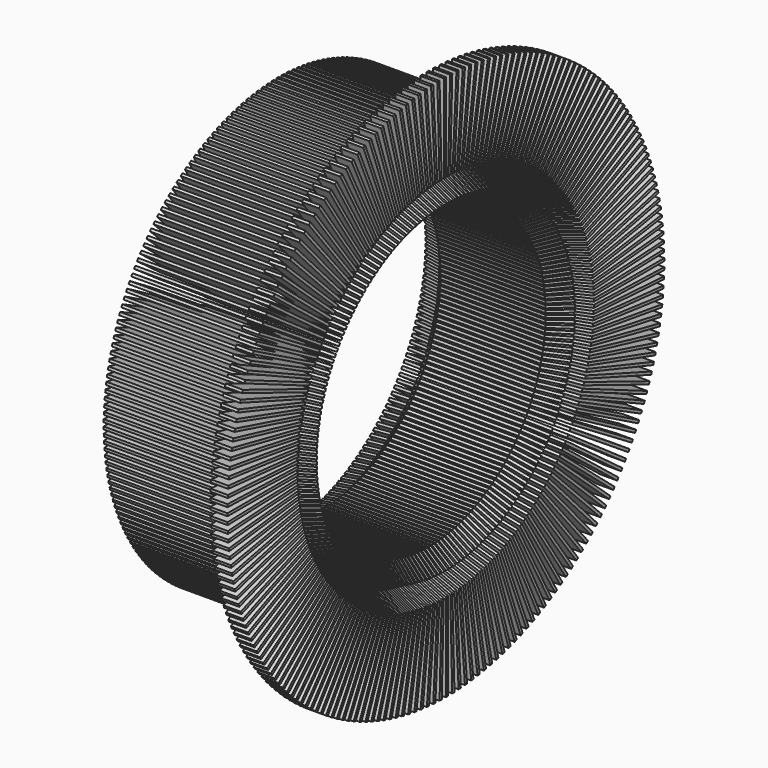
from build123d import *

# Parameters (mm, degrees)
F0_R     = 13
F1_DEPTH = 3
F2_COUNT = 216
F2_ANGLE = 358.333319


with BuildPart() as f1:
    # F0 (on Front) → F1 (new body)
    with BuildSketch(Plane.XZ):
        with BuildLine():
            Line((79.4218590744, 204.5887249741), (79.4218590744, 302.0993764614))
            Line((79.4218590744, 302.0993764614), (60.4218590744, 302.0993764614))
            Line((60.4218590744, 302.0993764614), (60.4218590744, 242.0993764614))
            ThreePointArc((60.4218590744, 242.0993764614), (55.8752099476, 238.8486342481), (51.3285608207, 242.0993764614))
            Line((51.3285608207, 242.0993764614), (-105.6314391793, 242.0993764614))
            Line((-105.6314391793, 242.0993764614), (-105.6314391793, 202.8593764614))
            Line((-105.6314391793, 202.8593764614), (-56.7432582628, 192.3738737706))
            Line((-56.7432582628, 192.3738737706), (-70.0419396162, 177.6219755411))
            Line((-70.0419396162, 177.6219755411), (-56.2349801763, 162))
            Line((-56.2349801763, 162), (60.158367424, 162))
            Line((60.158367424, 162), (79.4218590744, 178.5993582789))
            Line((79.4218590744, 178.5993582789), (52.476448941, 192.3738737706))
            Line((52.476448941, 192.3738737706), (79.4218590744, 204.5887249741))
        make_face()
        with Locations((5.6830663262, 192.3738737706)):
            Circle(F0_R, mode=Mode.SUBTRACT)
    extrude(amount=F1_DEPTH)


with BuildPart() as f2_1:
    # F2: instance of F1
    add(f1.part.rotate(Axis((24.8979143798, 0, 0), (1, 0, 0)), 1 * F2_ANGLE / (F2_COUNT - 1)))


with BuildPart() as f2_2:
    # F2: instance of F1
    add(f1.part.rotate(Axis((24.8979143798, 0, 0), (1, 0, 0)), 2 * F2_ANGLE / (F2_COUNT - 1)))


with BuildPart() as f2_3:
    # F2: instance of F1
    add(f1.part.rotate(Axis((24.8979143798, 0, 0), (1, 0, 0)), 3 * F2_ANGLE / (F2_COUNT - 1)))


with BuildPart() as f2_4:
    # F2: instance of F1
    add(f1.part.rotate(Axis((24.8979143798, 0, 0), (1, 0, 0)), 4 * F2_ANGLE / (F2_COUNT - 1)))


with BuildPart() as f2_5:
    # F2: instance of F1
    add(f1.part.rotate(Axis((24.8979143798, 0, 0), (1, 0, 0)), 5 * F2_ANGLE / (F2_COUNT - 1)))


with BuildPart() as f2_6:
    # F2: instance of F1
    add(f1.part.rotate(Axis((24.8979143798, 0, 0), (1, 0, 0)), 6 * F2_ANGLE / (F2_COUNT - 1)))


with BuildPart() as f2_7:
    # F2: instance of F1
    add(f1.part.rotate(Axis((24.8979143798, 0, 0), (1, 0, 0)), 7 * F2_ANGLE / (F2_COUNT - 1)))


with BuildPart() as f2_8:
    # F2: instance of F1
    add(f1.part.rotate(Axis((24.8979143798, 0, 0), (1, 0, 0)), 8 * F2_ANGLE / (F2_COUNT - 1)))


with BuildPart() as f2_9:
    # F2: instance of F1
    add(f1.part.rotate(Axis((24.8979143798, 0, 0), (1, 0, 0)), 9 * F2_ANGLE / (F2_COUNT - 1)))


with BuildPart() as f2_10:
    # F2: instance of F1
    add(f1.part.rotate(Axis((24.8979143798, 0, 0), (1, 0, 0)), 10 * F2_ANGLE / (F2_COUNT - 1)))


with BuildPart() as f2_11:
    # F2: instance of F1
    add(f1.part.rotate(Axis((24.8979143798, 0, 0), (1, 0, 0)), 11 * F2_ANGLE / (F2_COUNT - 1)))


with BuildPart() as f2_12:
    # F2: instance of F1
    add(f1.part.rotate(Axis((24.8979143798, 0, 0), (1, 0, 0)), 12 * F2_ANGLE / (F2_COUNT - 1)))


with BuildPart() as f2_13:
    # F2: instance of F1
    add(f1.part.rotate(Axis((24.8979143798, 0, 0), (1, 0, 0)), 13 * F2_ANGLE / (F2_COUNT - 1)))


with BuildPart() as f2_14:
    # F2: instance of F1
    add(f1.part.rotate(Axis((24.8979143798, 0, 0), (1, 0, 0)), 14 * F2_ANGLE / (F2_COUNT - 1)))


with BuildPart() as f2_15:
    # F2: instance of F1
    add(f1.part.rotate(Axis((24.8979143798, 0, 0), (1, 0, 0)), 15 * F2_ANGLE / (F2_COUNT - 1)))


with BuildPart() as f2_16:
    # F2: instance of F1
    add(f1.part.rotate(Axis((24.8979143798, 0, 0), (1, 0, 0)), 16 * F2_ANGLE / (F2_COUNT - 1)))


with BuildPart() as f2_17:
    # F2: instance of F1
    add(f1.part.rotate(Axis((24.8979143798, 0, 0), (1, 0, 0)), 17 * F2_ANGLE / (F2_COUNT - 1)))


with BuildPart() as f2_18:
    # F2: instance of F1
    add(f1.part.rotate(Axis((24.8979143798, 0, 0), (1, 0, 0)), 18 * F2_ANGLE / (F2_COUNT - 1)))


with BuildPart() as f2_19:
    # F2: instance of F1
    add(f1.part.rotate(Axis((24.8979143798, 0, 0), (1, 0, 0)), 19 * F2_ANGLE / (F2_COUNT - 1)))


with BuildPart() as f2_20:
    # F2: instance of F1
    add(f1.part.rotate(Axis((24.8979143798, 0, 0), (1, 0, 0)), 20 * F2_ANGLE / (F2_COUNT - 1)))


with BuildPart() as f2_21:
    # F2: instance of F1
    add(f1.part.rotate(Axis((24.8979143798, 0, 0), (1, 0, 0)), 21 * F2_ANGLE / (F2_COUNT - 1)))


with BuildPart() as f2_22:
    # F2: instance of F1
    add(f1.part.rotate(Axis((24.8979143798, 0, 0), (1, 0, 0)), 22 * F2_ANGLE / (F2_COUNT - 1)))


with BuildPart() as f2_23:
    # F2: instance of F1
    add(f1.part.rotate(Axis((24.8979143798, 0, 0), (1, 0, 0)), 23 * F2_ANGLE / (F2_COUNT - 1)))


with BuildPart() as f2_24:
    # F2: instance of F1
    add(f1.part.rotate(Axis((24.8979143798, 0, 0), (1, 0, 0)), 24 * F2_ANGLE / (F2_COUNT - 1)))


with BuildPart() as f2_25:
    # F2: instance of F1
    add(f1.part.rotate(Axis((24.8979143798, 0, 0), (1, 0, 0)), 25 * F2_ANGLE / (F2_COUNT - 1)))


with BuildPart() as f2_26:
    # F2: instance of F1
    add(f1.part.rotate(Axis((24.8979143798, 0, 0), (1, 0, 0)), 26 * F2_ANGLE / (F2_COUNT - 1)))


with BuildPart() as f2_27:
    # F2: instance of F1
    add(f1.part.rotate(Axis((24.8979143798, 0, 0), (1, 0, 0)), 27 * F2_ANGLE / (F2_COUNT - 1)))


with BuildPart() as f2_28:
    # F2: instance of F1
    add(f1.part.rotate(Axis((24.8979143798, 0, 0), (1, 0, 0)), 28 * F2_ANGLE / (F2_COUNT - 1)))


with BuildPart() as f2_29:
    # F2: instance of F1
    add(f1.part.rotate(Axis((24.8979143798, 0, 0), (1, 0, 0)), 29 * F2_ANGLE / (F2_COUNT - 1)))


with BuildPart() as f2_30:
    # F2: instance of F1
    add(f1.part.rotate(Axis((24.8979143798, 0, 0), (1, 0, 0)), 30 * F2_ANGLE / (F2_COUNT - 1)))


with BuildPart() as f2_31:
    # F2: instance of F1
    add(f1.part.rotate(Axis((24.8979143798, 0, 0), (1, 0, 0)), 31 * F2_ANGLE / (F2_COUNT - 1)))


with BuildPart() as f2_32:
    # F2: instance of F1
    add(f1.part.rotate(Axis((24.8979143798, 0, 0), (1, 0, 0)), 32 * F2_ANGLE / (F2_COUNT - 1)))


with BuildPart() as f2_33:
    # F2: instance of F1
    add(f1.part.rotate(Axis((24.8979143798, 0, 0), (1, 0, 0)), 33 * F2_ANGLE / (F2_COUNT - 1)))


with BuildPart() as f2_34:
    # F2: instance of F1
    add(f1.part.rotate(Axis((24.8979143798, 0, 0), (1, 0, 0)), 34 * F2_ANGLE / (F2_COUNT - 1)))


with BuildPart() as f2_35:
    # F2: instance of F1
    add(f1.part.rotate(Axis((24.8979143798, 0, 0), (1, 0, 0)), 35 * F2_ANGLE / (F2_COUNT - 1)))


with BuildPart() as f2_36:
    # F2: instance of F1
    add(f1.part.rotate(Axis((24.8979143798, 0, 0), (1, 0, 0)), 36 * F2_ANGLE / (F2_COUNT - 1)))


with BuildPart() as f2_37:
    # F2: instance of F1
    add(f1.part.rotate(Axis((24.8979143798, 0, 0), (1, 0, 0)), 37 * F2_ANGLE / (F2_COUNT - 1)))


with BuildPart() as f2_38:
    # F2: instance of F1
    add(f1.part.rotate(Axis((24.8979143798, 0, 0), (1, 0, 0)), 38 * F2_ANGLE / (F2_COUNT - 1)))


with BuildPart() as f2_39:
    # F2: instance of F1
    add(f1.part.rotate(Axis((24.8979143798, 0, 0), (1, 0, 0)), 39 * F2_ANGLE / (F2_COUNT - 1)))


with BuildPart() as f2_40:
    # F2: instance of F1
    add(f1.part.rotate(Axis((24.8979143798, 0, 0), (1, 0, 0)), 40 * F2_ANGLE / (F2_COUNT - 1)))


with BuildPart() as f2_41:
    # F2: instance of F1
    add(f1.part.rotate(Axis((24.8979143798, 0, 0), (1, 0, 0)), 41 * F2_ANGLE / (F2_COUNT - 1)))


with BuildPart() as f2_42:
    # F2: instance of F1
    add(f1.part.rotate(Axis((24.8979143798, 0, 0), (1, 0, 0)), 42 * F2_ANGLE / (F2_COUNT - 1)))


with BuildPart() as f2_43:
    # F2: instance of F1
    add(f1.part.rotate(Axis((24.8979143798, 0, 0), (1, 0, 0)), 43 * F2_ANGLE / (F2_COUNT - 1)))


with BuildPart() as f2_44:
    # F2: instance of F1
    add(f1.part.rotate(Axis((24.8979143798, 0, 0), (1, 0, 0)), 44 * F2_ANGLE / (F2_COUNT - 1)))


with BuildPart() as f2_45:
    # F2: instance of F1
    add(f1.part.rotate(Axis((24.8979143798, 0, 0), (1, 0, 0)), 45 * F2_ANGLE / (F2_COUNT - 1)))


with BuildPart() as f2_46:
    # F2: instance of F1
    add(f1.part.rotate(Axis((24.8979143798, 0, 0), (1, 0, 0)), 46 * F2_ANGLE / (F2_COUNT - 1)))


with BuildPart() as f2_47:
    # F2: instance of F1
    add(f1.part.rotate(Axis((24.8979143798, 0, 0), (1, 0, 0)), 47 * F2_ANGLE / (F2_COUNT - 1)))


with BuildPart() as f2_48:
    # F2: instance of F1
    add(f1.part.rotate(Axis((24.8979143798, 0, 0), (1, 0, 0)), 48 * F2_ANGLE / (F2_COUNT - 1)))


with BuildPart() as f2_49:
    # F2: instance of F1
    add(f1.part.rotate(Axis((24.8979143798, 0, 0), (1, 0, 0)), 49 * F2_ANGLE / (F2_COUNT - 1)))


with BuildPart() as f2_50:
    # F2: instance of F1
    add(f1.part.rotate(Axis((24.8979143798, 0, 0), (1, 0, 0)), 50 * F2_ANGLE / (F2_COUNT - 1)))


with BuildPart() as f2_51:
    # F2: instance of F1
    add(f1.part.rotate(Axis((24.8979143798, 0, 0), (1, 0, 0)), 51 * F2_ANGLE / (F2_COUNT - 1)))


with BuildPart() as f2_52:
    # F2: instance of F1
    add(f1.part.rotate(Axis((24.8979143798, 0, 0), (1, 0, 0)), 52 * F2_ANGLE / (F2_COUNT - 1)))


with BuildPart() as f2_53:
    # F2: instance of F1
    add(f1.part.rotate(Axis((24.8979143798, 0, 0), (1, 0, 0)), 53 * F2_ANGLE / (F2_COUNT - 1)))


with BuildPart() as f2_54:
    # F2: instance of F1
    add(f1.part.rotate(Axis((24.8979143798, 0, 0), (1, 0, 0)), 54 * F2_ANGLE / (F2_COUNT - 1)))


with BuildPart() as f2_55:
    # F2: instance of F1
    add(f1.part.rotate(Axis((24.8979143798, 0, 0), (1, 0, 0)), 55 * F2_ANGLE / (F2_COUNT - 1)))


with BuildPart() as f2_56:
    # F2: instance of F1
    add(f1.part.rotate(Axis((24.8979143798, 0, 0), (1, 0, 0)), 56 * F2_ANGLE / (F2_COUNT - 1)))


with BuildPart() as f2_57:
    # F2: instance of F1
    add(f1.part.rotate(Axis((24.8979143798, 0, 0), (1, 0, 0)), 57 * F2_ANGLE / (F2_COUNT - 1)))


with BuildPart() as f2_58:
    # F2: instance of F1
    add(f1.part.rotate(Axis((24.8979143798, 0, 0), (1, 0, 0)), 58 * F2_ANGLE / (F2_COUNT - 1)))


with BuildPart() as f2_59:
    # F2: instance of F1
    add(f1.part.rotate(Axis((24.8979143798, 0, 0), (1, 0, 0)), 59 * F2_ANGLE / (F2_COUNT - 1)))


with BuildPart() as f2_60:
    # F2: instance of F1
    add(f1.part.rotate(Axis((24.8979143798, 0, 0), (1, 0, 0)), 60 * F2_ANGLE / (F2_COUNT - 1)))


with BuildPart() as f2_61:
    # F2: instance of F1
    add(f1.part.rotate(Axis((24.8979143798, 0, 0), (1, 0, 0)), 61 * F2_ANGLE / (F2_COUNT - 1)))


with BuildPart() as f2_62:
    # F2: instance of F1
    add(f1.part.rotate(Axis((24.8979143798, 0, 0), (1, 0, 0)), 62 * F2_ANGLE / (F2_COUNT - 1)))


with BuildPart() as f2_63:
    # F2: instance of F1
    add(f1.part.rotate(Axis((24.8979143798, 0, 0), (1, 0, 0)), 63 * F2_ANGLE / (F2_COUNT - 1)))


with BuildPart() as f2_64:
    # F2: instance of F1
    add(f1.part.rotate(Axis((24.8979143798, 0, 0), (1, 0, 0)), 64 * F2_ANGLE / (F2_COUNT - 1)))


with BuildPart() as f2_65:
    # F2: instance of F1
    add(f1.part.rotate(Axis((24.8979143798, 0, 0), (1, 0, 0)), 65 * F2_ANGLE / (F2_COUNT - 1)))


with BuildPart() as f2_66:
    # F2: instance of F1
    add(f1.part.rotate(Axis((24.8979143798, 0, 0), (1, 0, 0)), 66 * F2_ANGLE / (F2_COUNT - 1)))


with BuildPart() as f2_67:
    # F2: instance of F1
    add(f1.part.rotate(Axis((24.8979143798, 0, 0), (1, 0, 0)), 67 * F2_ANGLE / (F2_COUNT - 1)))


with BuildPart() as f2_68:
    # F2: instance of F1
    add(f1.part.rotate(Axis((24.8979143798, 0, 0), (1, 0, 0)), 68 * F2_ANGLE / (F2_COUNT - 1)))


with BuildPart() as f2_69:
    # F2: instance of F1
    add(f1.part.rotate(Axis((24.8979143798, 0, 0), (1, 0, 0)), 69 * F2_ANGLE / (F2_COUNT - 1)))


with BuildPart() as f2_70:
    # F2: instance of F1
    add(f1.part.rotate(Axis((24.8979143798, 0, 0), (1, 0, 0)), 70 * F2_ANGLE / (F2_COUNT - 1)))


with BuildPart() as f2_71:
    # F2: instance of F1
    add(f1.part.rotate(Axis((24.8979143798, 0, 0), (1, 0, 0)), 71 * F2_ANGLE / (F2_COUNT - 1)))


with BuildPart() as f2_72:
    # F2: instance of F1
    add(f1.part.rotate(Axis((24.8979143798, 0, 0), (1, 0, 0)), 72 * F2_ANGLE / (F2_COUNT - 1)))


with BuildPart() as f2_73:
    # F2: instance of F1
    add(f1.part.rotate(Axis((24.8979143798, 0, 0), (1, 0, 0)), 73 * F2_ANGLE / (F2_COUNT - 1)))


with BuildPart() as f2_74:
    # F2: instance of F1
    add(f1.part.rotate(Axis((24.8979143798, 0, 0), (1, 0, 0)), 74 * F2_ANGLE / (F2_COUNT - 1)))


with BuildPart() as f2_75:
    # F2: instance of F1
    add(f1.part.rotate(Axis((24.8979143798, 0, 0), (1, 0, 0)), 75 * F2_ANGLE / (F2_COUNT - 1)))


with BuildPart() as f2_76:
    # F2: instance of F1
    add(f1.part.rotate(Axis((24.8979143798, 0, 0), (1, 0, 0)), 76 * F2_ANGLE / (F2_COUNT - 1)))


with BuildPart() as f2_77:
    # F2: instance of F1
    add(f1.part.rotate(Axis((24.8979143798, 0, 0), (1, 0, 0)), 77 * F2_ANGLE / (F2_COUNT - 1)))


with BuildPart() as f2_78:
    # F2: instance of F1
    add(f1.part.rotate(Axis((24.8979143798, 0, 0), (1, 0, 0)), 78 * F2_ANGLE / (F2_COUNT - 1)))


with BuildPart() as f2_79:
    # F2: instance of F1
    add(f1.part.rotate(Axis((24.8979143798, 0, 0), (1, 0, 0)), 79 * F2_ANGLE / (F2_COUNT - 1)))


with BuildPart() as f2_80:
    # F2: instance of F1
    add(f1.part.rotate(Axis((24.8979143798, 0, 0), (1, 0, 0)), 80 * F2_ANGLE / (F2_COUNT - 1)))


with BuildPart() as f2_81:
    # F2: instance of F1
    add(f1.part.rotate(Axis((24.8979143798, 0, 0), (1, 0, 0)), 81 * F2_ANGLE / (F2_COUNT - 1)))


with BuildPart() as f2_82:
    # F2: instance of F1
    add(f1.part.rotate(Axis((24.8979143798, 0, 0), (1, 0, 0)), 82 * F2_ANGLE / (F2_COUNT - 1)))


with BuildPart() as f2_83:
    # F2: instance of F1
    add(f1.part.rotate(Axis((24.8979143798, 0, 0), (1, 0, 0)), 83 * F2_ANGLE / (F2_COUNT - 1)))


with BuildPart() as f2_84:
    # F2: instance of F1
    add(f1.part.rotate(Axis((24.8979143798, 0, 0), (1, 0, 0)), 84 * F2_ANGLE / (F2_COUNT - 1)))


with BuildPart() as f2_85:
    # F2: instance of F1
    add(f1.part.rotate(Axis((24.8979143798, 0, 0), (1, 0, 0)), 85 * F2_ANGLE / (F2_COUNT - 1)))


with BuildPart() as f2_86:
    # F2: instance of F1
    add(f1.part.rotate(Axis((24.8979143798, 0, 0), (1, 0, 0)), 86 * F2_ANGLE / (F2_COUNT - 1)))


with BuildPart() as f2_87:
    # F2: instance of F1
    add(f1.part.rotate(Axis((24.8979143798, 0, 0), (1, 0, 0)), 87 * F2_ANGLE / (F2_COUNT - 1)))


with BuildPart() as f2_88:
    # F2: instance of F1
    add(f1.part.rotate(Axis((24.8979143798, 0, 0), (1, 0, 0)), 88 * F2_ANGLE / (F2_COUNT - 1)))


with BuildPart() as f2_89:
    # F2: instance of F1
    add(f1.part.rotate(Axis((24.8979143798, 0, 0), (1, 0, 0)), 89 * F2_ANGLE / (F2_COUNT - 1)))


with BuildPart() as f2_90:
    # F2: instance of F1
    add(f1.part.rotate(Axis((24.8979143798, 0, 0), (1, 0, 0)), 90 * F2_ANGLE / (F2_COUNT - 1)))


with BuildPart() as f2_91:
    # F2: instance of F1
    add(f1.part.rotate(Axis((24.8979143798, 0, 0), (1, 0, 0)), 91 * F2_ANGLE / (F2_COUNT - 1)))


with BuildPart() as f2_92:
    # F2: instance of F1
    add(f1.part.rotate(Axis((24.8979143798, 0, 0), (1, 0, 0)), 92 * F2_ANGLE / (F2_COUNT - 1)))


with BuildPart() as f2_93:
    # F2: instance of F1
    add(f1.part.rotate(Axis((24.8979143798, 0, 0), (1, 0, 0)), 93 * F2_ANGLE / (F2_COUNT - 1)))


with BuildPart() as f2_94:
    # F2: instance of F1
    add(f1.part.rotate(Axis((24.8979143798, 0, 0), (1, 0, 0)), 94 * F2_ANGLE / (F2_COUNT - 1)))


with BuildPart() as f2_95:
    # F2: instance of F1
    add(f1.part.rotate(Axis((24.8979143798, 0, 0), (1, 0, 0)), 95 * F2_ANGLE / (F2_COUNT - 1)))


with BuildPart() as f2_96:
    # F2: instance of F1
    add(f1.part.rotate(Axis((24.8979143798, 0, 0), (1, 0, 0)), 96 * F2_ANGLE / (F2_COUNT - 1)))


with BuildPart() as f2_97:
    # F2: instance of F1
    add(f1.part.rotate(Axis((24.8979143798, 0, 0), (1, 0, 0)), 97 * F2_ANGLE / (F2_COUNT - 1)))


with BuildPart() as f2_98:
    # F2: instance of F1
    add(f1.part.rotate(Axis((24.8979143798, 0, 0), (1, 0, 0)), 98 * F2_ANGLE / (F2_COUNT - 1)))


with BuildPart() as f2_99:
    # F2: instance of F1
    add(f1.part.rotate(Axis((24.8979143798, 0, 0), (1, 0, 0)), 99 * F2_ANGLE / (F2_COUNT - 1)))


with BuildPart() as f2_100:
    # F2: instance of F1
    add(f1.part.rotate(Axis((24.8979143798, 0, 0), (1, 0, 0)), 100 * F2_ANGLE / (F2_COUNT - 1)))


with BuildPart() as f2_101:
    # F2: instance of F1
    add(f1.part.rotate(Axis((24.8979143798, 0, 0), (1, 0, 0)), 101 * F2_ANGLE / (F2_COUNT - 1)))


with BuildPart() as f2_102:
    # F2: instance of F1
    add(f1.part.rotate(Axis((24.8979143798, 0, 0), (1, 0, 0)), 102 * F2_ANGLE / (F2_COUNT - 1)))


with BuildPart() as f2_103:
    # F2: instance of F1
    add(f1.part.rotate(Axis((24.8979143798, 0, 0), (1, 0, 0)), 103 * F2_ANGLE / (F2_COUNT - 1)))


with BuildPart() as f2_104:
    # F2: instance of F1
    add(f1.part.rotate(Axis((24.8979143798, 0, 0), (1, 0, 0)), 104 * F2_ANGLE / (F2_COUNT - 1)))


with BuildPart() as f2_105:
    # F2: instance of F1
    add(f1.part.rotate(Axis((24.8979143798, 0, 0), (1, 0, 0)), 105 * F2_ANGLE / (F2_COUNT - 1)))


with BuildPart() as f2_106:
    # F2: instance of F1
    add(f1.part.rotate(Axis((24.8979143798, 0, 0), (1, 0, 0)), 106 * F2_ANGLE / (F2_COUNT - 1)))


with BuildPart() as f2_107:
    # F2: instance of F1
    add(f1.part.rotate(Axis((24.8979143798, 0, 0), (1, 0, 0)), 107 * F2_ANGLE / (F2_COUNT - 1)))


with BuildPart() as f2_108:
    # F2: instance of F1
    add(f1.part.rotate(Axis((24.8979143798, 0, 0), (1, 0, 0)), 108 * F2_ANGLE / (F2_COUNT - 1)))


with BuildPart() as f2_109:
    # F2: instance of F1
    add(f1.part.rotate(Axis((24.8979143798, 0, 0), (1, 0, 0)), 109 * F2_ANGLE / (F2_COUNT - 1)))


with BuildPart() as f2_110:
    # F2: instance of F1
    add(f1.part.rotate(Axis((24.8979143798, 0, 0), (1, 0, 0)), 110 * F2_ANGLE / (F2_COUNT - 1)))


with BuildPart() as f2_111:
    # F2: instance of F1
    add(f1.part.rotate(Axis((24.8979143798, 0, 0), (1, 0, 0)), 111 * F2_ANGLE / (F2_COUNT - 1)))


with BuildPart() as f2_112:
    # F2: instance of F1
    add(f1.part.rotate(Axis((24.8979143798, 0, 0), (1, 0, 0)), 112 * F2_ANGLE / (F2_COUNT - 1)))


with BuildPart() as f2_113:
    # F2: instance of F1
    add(f1.part.rotate(Axis((24.8979143798, 0, 0), (1, 0, 0)), 113 * F2_ANGLE / (F2_COUNT - 1)))


with BuildPart() as f2_114:
    # F2: instance of F1
    add(f1.part.rotate(Axis((24.8979143798, 0, 0), (1, 0, 0)), 114 * F2_ANGLE / (F2_COUNT - 1)))


with BuildPart() as f2_115:
    # F2: instance of F1
    add(f1.part.rotate(Axis((24.8979143798, 0, 0), (1, 0, 0)), 115 * F2_ANGLE / (F2_COUNT - 1)))


with BuildPart() as f2_116:
    # F2: instance of F1
    add(f1.part.rotate(Axis((24.8979143798, 0, 0), (1, 0, 0)), 116 * F2_ANGLE / (F2_COUNT - 1)))


with BuildPart() as f2_117:
    # F2: instance of F1
    add(f1.part.rotate(Axis((24.8979143798, 0, 0), (1, 0, 0)), 117 * F2_ANGLE / (F2_COUNT - 1)))


with BuildPart() as f2_118:
    # F2: instance of F1
    add(f1.part.rotate(Axis((24.8979143798, 0, 0), (1, 0, 0)), 118 * F2_ANGLE / (F2_COUNT - 1)))


with BuildPart() as f2_119:
    # F2: instance of F1
    add(f1.part.rotate(Axis((24.8979143798, 0, 0), (1, 0, 0)), 119 * F2_ANGLE / (F2_COUNT - 1)))


with BuildPart() as f2_120:
    # F2: instance of F1
    add(f1.part.rotate(Axis((24.8979143798, 0, 0), (1, 0, 0)), 120 * F2_ANGLE / (F2_COUNT - 1)))


with BuildPart() as f2_121:
    # F2: instance of F1
    add(f1.part.rotate(Axis((24.8979143798, 0, 0), (1, 0, 0)), 121 * F2_ANGLE / (F2_COUNT - 1)))


with BuildPart() as f2_122:
    # F2: instance of F1
    add(f1.part.rotate(Axis((24.8979143798, 0, 0), (1, 0, 0)), 122 * F2_ANGLE / (F2_COUNT - 1)))


with BuildPart() as f2_123:
    # F2: instance of F1
    add(f1.part.rotate(Axis((24.8979143798, 0, 0), (1, 0, 0)), 123 * F2_ANGLE / (F2_COUNT - 1)))


with BuildPart() as f2_124:
    # F2: instance of F1
    add(f1.part.rotate(Axis((24.8979143798, 0, 0), (1, 0, 0)), 124 * F2_ANGLE / (F2_COUNT - 1)))


with BuildPart() as f2_125:
    # F2: instance of F1
    add(f1.part.rotate(Axis((24.8979143798, 0, 0), (1, 0, 0)), 125 * F2_ANGLE / (F2_COUNT - 1)))


with BuildPart() as f2_126:
    # F2: instance of F1
    add(f1.part.rotate(Axis((24.8979143798, 0, 0), (1, 0, 0)), 126 * F2_ANGLE / (F2_COUNT - 1)))


with BuildPart() as f2_127:
    # F2: instance of F1
    add(f1.part.rotate(Axis((24.8979143798, 0, 0), (1, 0, 0)), 127 * F2_ANGLE / (F2_COUNT - 1)))


with BuildPart() as f2_128:
    # F2: instance of F1
    add(f1.part.rotate(Axis((24.8979143798, 0, 0), (1, 0, 0)), 128 * F2_ANGLE / (F2_COUNT - 1)))


with BuildPart() as f2_129:
    # F2: instance of F1
    add(f1.part.rotate(Axis((24.8979143798, 0, 0), (1, 0, 0)), 129 * F2_ANGLE / (F2_COUNT - 1)))


with BuildPart() as f2_130:
    # F2: instance of F1
    add(f1.part.rotate(Axis((24.8979143798, 0, 0), (1, 0, 0)), 130 * F2_ANGLE / (F2_COUNT - 1)))


with BuildPart() as f2_131:
    # F2: instance of F1
    add(f1.part.rotate(Axis((24.8979143798, 0, 0), (1, 0, 0)), 131 * F2_ANGLE / (F2_COUNT - 1)))


with BuildPart() as f2_132:
    # F2: instance of F1
    add(f1.part.rotate(Axis((24.8979143798, 0, 0), (1, 0, 0)), 132 * F2_ANGLE / (F2_COUNT - 1)))


with BuildPart() as f2_133:
    # F2: instance of F1
    add(f1.part.rotate(Axis((24.8979143798, 0, 0), (1, 0, 0)), 133 * F2_ANGLE / (F2_COUNT - 1)))


with BuildPart() as f2_134:
    # F2: instance of F1
    add(f1.part.rotate(Axis((24.8979143798, 0, 0), (1, 0, 0)), 134 * F2_ANGLE / (F2_COUNT - 1)))


with BuildPart() as f2_135:
    # F2: instance of F1
    add(f1.part.rotate(Axis((24.8979143798, 0, 0), (1, 0, 0)), 135 * F2_ANGLE / (F2_COUNT - 1)))


with BuildPart() as f2_136:
    # F2: instance of F1
    add(f1.part.rotate(Axis((24.8979143798, 0, 0), (1, 0, 0)), 136 * F2_ANGLE / (F2_COUNT - 1)))


with BuildPart() as f2_137:
    # F2: instance of F1
    add(f1.part.rotate(Axis((24.8979143798, 0, 0), (1, 0, 0)), 137 * F2_ANGLE / (F2_COUNT - 1)))


with BuildPart() as f2_138:
    # F2: instance of F1
    add(f1.part.rotate(Axis((24.8979143798, 0, 0), (1, 0, 0)), 138 * F2_ANGLE / (F2_COUNT - 1)))


with BuildPart() as f2_139:
    # F2: instance of F1
    add(f1.part.rotate(Axis((24.8979143798, 0, 0), (1, 0, 0)), 139 * F2_ANGLE / (F2_COUNT - 1)))


with BuildPart() as f2_140:
    # F2: instance of F1
    add(f1.part.rotate(Axis((24.8979143798, 0, 0), (1, 0, 0)), 140 * F2_ANGLE / (F2_COUNT - 1)))


with BuildPart() as f2_141:
    # F2: instance of F1
    add(f1.part.rotate(Axis((24.8979143798, 0, 0), (1, 0, 0)), 141 * F2_ANGLE / (F2_COUNT - 1)))


with BuildPart() as f2_142:
    # F2: instance of F1
    add(f1.part.rotate(Axis((24.8979143798, 0, 0), (1, 0, 0)), 142 * F2_ANGLE / (F2_COUNT - 1)))


with BuildPart() as f2_143:
    # F2: instance of F1
    add(f1.part.rotate(Axis((24.8979143798, 0, 0), (1, 0, 0)), 143 * F2_ANGLE / (F2_COUNT - 1)))


with BuildPart() as f2_144:
    # F2: instance of F1
    add(f1.part.rotate(Axis((24.8979143798, 0, 0), (1, 0, 0)), 144 * F2_ANGLE / (F2_COUNT - 1)))


with BuildPart() as f2_145:
    # F2: instance of F1
    add(f1.part.rotate(Axis((24.8979143798, 0, 0), (1, 0, 0)), 145 * F2_ANGLE / (F2_COUNT - 1)))


with BuildPart() as f2_146:
    # F2: instance of F1
    add(f1.part.rotate(Axis((24.8979143798, 0, 0), (1, 0, 0)), 146 * F2_ANGLE / (F2_COUNT - 1)))


with BuildPart() as f2_147:
    # F2: instance of F1
    add(f1.part.rotate(Axis((24.8979143798, 0, 0), (1, 0, 0)), 147 * F2_ANGLE / (F2_COUNT - 1)))


with BuildPart() as f2_148:
    # F2: instance of F1
    add(f1.part.rotate(Axis((24.8979143798, 0, 0), (1, 0, 0)), 148 * F2_ANGLE / (F2_COUNT - 1)))


with BuildPart() as f2_149:
    # F2: instance of F1
    add(f1.part.rotate(Axis((24.8979143798, 0, 0), (1, 0, 0)), 149 * F2_ANGLE / (F2_COUNT - 1)))


with BuildPart() as f2_150:
    # F2: instance of F1
    add(f1.part.rotate(Axis((24.8979143798, 0, 0), (1, 0, 0)), 150 * F2_ANGLE / (F2_COUNT - 1)))


with BuildPart() as f2_151:
    # F2: instance of F1
    add(f1.part.rotate(Axis((24.8979143798, 0, 0), (1, 0, 0)), 151 * F2_ANGLE / (F2_COUNT - 1)))


with BuildPart() as f2_152:
    # F2: instance of F1
    add(f1.part.rotate(Axis((24.8979143798, 0, 0), (1, 0, 0)), 152 * F2_ANGLE / (F2_COUNT - 1)))


with BuildPart() as f2_153:
    # F2: instance of F1
    add(f1.part.rotate(Axis((24.8979143798, 0, 0), (1, 0, 0)), 153 * F2_ANGLE / (F2_COUNT - 1)))


with BuildPart() as f2_154:
    # F2: instance of F1
    add(f1.part.rotate(Axis((24.8979143798, 0, 0), (1, 0, 0)), 154 * F2_ANGLE / (F2_COUNT - 1)))


with BuildPart() as f2_155:
    # F2: instance of F1
    add(f1.part.rotate(Axis((24.8979143798, 0, 0), (1, 0, 0)), 155 * F2_ANGLE / (F2_COUNT - 1)))


with BuildPart() as f2_156:
    # F2: instance of F1
    add(f1.part.rotate(Axis((24.8979143798, 0, 0), (1, 0, 0)), 156 * F2_ANGLE / (F2_COUNT - 1)))


with BuildPart() as f2_157:
    # F2: instance of F1
    add(f1.part.rotate(Axis((24.8979143798, 0, 0), (1, 0, 0)), 157 * F2_ANGLE / (F2_COUNT - 1)))


with BuildPart() as f2_158:
    # F2: instance of F1
    add(f1.part.rotate(Axis((24.8979143798, 0, 0), (1, 0, 0)), 158 * F2_ANGLE / (F2_COUNT - 1)))


with BuildPart() as f2_159:
    # F2: instance of F1
    add(f1.part.rotate(Axis((24.8979143798, 0, 0), (1, 0, 0)), 159 * F2_ANGLE / (F2_COUNT - 1)))


with BuildPart() as f2_160:
    # F2: instance of F1
    add(f1.part.rotate(Axis((24.8979143798, 0, 0), (1, 0, 0)), 160 * F2_ANGLE / (F2_COUNT - 1)))


with BuildPart() as f2_161:
    # F2: instance of F1
    add(f1.part.rotate(Axis((24.8979143798, 0, 0), (1, 0, 0)), 161 * F2_ANGLE / (F2_COUNT - 1)))


with BuildPart() as f2_162:
    # F2: instance of F1
    add(f1.part.rotate(Axis((24.8979143798, 0, 0), (1, 0, 0)), 162 * F2_ANGLE / (F2_COUNT - 1)))


with BuildPart() as f2_163:
    # F2: instance of F1
    add(f1.part.rotate(Axis((24.8979143798, 0, 0), (1, 0, 0)), 163 * F2_ANGLE / (F2_COUNT - 1)))


with BuildPart() as f2_164:
    # F2: instance of F1
    add(f1.part.rotate(Axis((24.8979143798, 0, 0), (1, 0, 0)), 164 * F2_ANGLE / (F2_COUNT - 1)))


with BuildPart() as f2_165:
    # F2: instance of F1
    add(f1.part.rotate(Axis((24.8979143798, 0, 0), (1, 0, 0)), 165 * F2_ANGLE / (F2_COUNT - 1)))


with BuildPart() as f2_166:
    # F2: instance of F1
    add(f1.part.rotate(Axis((24.8979143798, 0, 0), (1, 0, 0)), 166 * F2_ANGLE / (F2_COUNT - 1)))


with BuildPart() as f2_167:
    # F2: instance of F1
    add(f1.part.rotate(Axis((24.8979143798, 0, 0), (1, 0, 0)), 167 * F2_ANGLE / (F2_COUNT - 1)))


with BuildPart() as f2_168:
    # F2: instance of F1
    add(f1.part.rotate(Axis((24.8979143798, 0, 0), (1, 0, 0)), 168 * F2_ANGLE / (F2_COUNT - 1)))


with BuildPart() as f2_169:
    # F2: instance of F1
    add(f1.part.rotate(Axis((24.8979143798, 0, 0), (1, 0, 0)), 169 * F2_ANGLE / (F2_COUNT - 1)))


with BuildPart() as f2_170:
    # F2: instance of F1
    add(f1.part.rotate(Axis((24.8979143798, 0, 0), (1, 0, 0)), 170 * F2_ANGLE / (F2_COUNT - 1)))


with BuildPart() as f2_171:
    # F2: instance of F1
    add(f1.part.rotate(Axis((24.8979143798, 0, 0), (1, 0, 0)), 171 * F2_ANGLE / (F2_COUNT - 1)))


with BuildPart() as f2_172:
    # F2: instance of F1
    add(f1.part.rotate(Axis((24.8979143798, 0, 0), (1, 0, 0)), 172 * F2_ANGLE / (F2_COUNT - 1)))


with BuildPart() as f2_173:
    # F2: instance of F1
    add(f1.part.rotate(Axis((24.8979143798, 0, 0), (1, 0, 0)), 173 * F2_ANGLE / (F2_COUNT - 1)))


with BuildPart() as f2_174:
    # F2: instance of F1
    add(f1.part.rotate(Axis((24.8979143798, 0, 0), (1, 0, 0)), 174 * F2_ANGLE / (F2_COUNT - 1)))


with BuildPart() as f2_175:
    # F2: instance of F1
    add(f1.part.rotate(Axis((24.8979143798, 0, 0), (1, 0, 0)), 175 * F2_ANGLE / (F2_COUNT - 1)))


with BuildPart() as f2_176:
    # F2: instance of F1
    add(f1.part.rotate(Axis((24.8979143798, 0, 0), (1, 0, 0)), 176 * F2_ANGLE / (F2_COUNT - 1)))


with BuildPart() as f2_177:
    # F2: instance of F1
    add(f1.part.rotate(Axis((24.8979143798, 0, 0), (1, 0, 0)), 177 * F2_ANGLE / (F2_COUNT - 1)))


with BuildPart() as f2_178:
    # F2: instance of F1
    add(f1.part.rotate(Axis((24.8979143798, 0, 0), (1, 0, 0)), 178 * F2_ANGLE / (F2_COUNT - 1)))


with BuildPart() as f2_179:
    # F2: instance of F1
    add(f1.part.rotate(Axis((24.8979143798, 0, 0), (1, 0, 0)), 179 * F2_ANGLE / (F2_COUNT - 1)))


with BuildPart() as f2_180:
    # F2: instance of F1
    add(f1.part.rotate(Axis((24.8979143798, 0, 0), (1, 0, 0)), 180 * F2_ANGLE / (F2_COUNT - 1)))


with BuildPart() as f2_181:
    # F2: instance of F1
    add(f1.part.rotate(Axis((24.8979143798, 0, 0), (1, 0, 0)), 181 * F2_ANGLE / (F2_COUNT - 1)))


with BuildPart() as f2_182:
    # F2: instance of F1
    add(f1.part.rotate(Axis((24.8979143798, 0, 0), (1, 0, 0)), 182 * F2_ANGLE / (F2_COUNT - 1)))


with BuildPart() as f2_183:
    # F2: instance of F1
    add(f1.part.rotate(Axis((24.8979143798, 0, 0), (1, 0, 0)), 183 * F2_ANGLE / (F2_COUNT - 1)))


with BuildPart() as f2_184:
    # F2: instance of F1
    add(f1.part.rotate(Axis((24.8979143798, 0, 0), (1, 0, 0)), 184 * F2_ANGLE / (F2_COUNT - 1)))


with BuildPart() as f2_185:
    # F2: instance of F1
    add(f1.part.rotate(Axis((24.8979143798, 0, 0), (1, 0, 0)), 185 * F2_ANGLE / (F2_COUNT - 1)))


with BuildPart() as f2_186:
    # F2: instance of F1
    add(f1.part.rotate(Axis((24.8979143798, 0, 0), (1, 0, 0)), 186 * F2_ANGLE / (F2_COUNT - 1)))


with BuildPart() as f2_187:
    # F2: instance of F1
    add(f1.part.rotate(Axis((24.8979143798, 0, 0), (1, 0, 0)), 187 * F2_ANGLE / (F2_COUNT - 1)))


with BuildPart() as f2_188:
    # F2: instance of F1
    add(f1.part.rotate(Axis((24.8979143798, 0, 0), (1, 0, 0)), 188 * F2_ANGLE / (F2_COUNT - 1)))


with BuildPart() as f2_189:
    # F2: instance of F1
    add(f1.part.rotate(Axis((24.8979143798, 0, 0), (1, 0, 0)), 189 * F2_ANGLE / (F2_COUNT - 1)))


with BuildPart() as f2_190:
    # F2: instance of F1
    add(f1.part.rotate(Axis((24.8979143798, 0, 0), (1, 0, 0)), 190 * F2_ANGLE / (F2_COUNT - 1)))


with BuildPart() as f2_191:
    # F2: instance of F1
    add(f1.part.rotate(Axis((24.8979143798, 0, 0), (1, 0, 0)), 191 * F2_ANGLE / (F2_COUNT - 1)))


with BuildPart() as f2_192:
    # F2: instance of F1
    add(f1.part.rotate(Axis((24.8979143798, 0, 0), (1, 0, 0)), 192 * F2_ANGLE / (F2_COUNT - 1)))


with BuildPart() as f2_193:
    # F2: instance of F1
    add(f1.part.rotate(Axis((24.8979143798, 0, 0), (1, 0, 0)), 193 * F2_ANGLE / (F2_COUNT - 1)))


with BuildPart() as f2_194:
    # F2: instance of F1
    add(f1.part.rotate(Axis((24.8979143798, 0, 0), (1, 0, 0)), 194 * F2_ANGLE / (F2_COUNT - 1)))


with BuildPart() as f2_195:
    # F2: instance of F1
    add(f1.part.rotate(Axis((24.8979143798, 0, 0), (1, 0, 0)), 195 * F2_ANGLE / (F2_COUNT - 1)))


with BuildPart() as f2_196:
    # F2: instance of F1
    add(f1.part.rotate(Axis((24.8979143798, 0, 0), (1, 0, 0)), 196 * F2_ANGLE / (F2_COUNT - 1)))


with BuildPart() as f2_197:
    # F2: instance of F1
    add(f1.part.rotate(Axis((24.8979143798, 0, 0), (1, 0, 0)), 197 * F2_ANGLE / (F2_COUNT - 1)))


with BuildPart() as f2_198:
    # F2: instance of F1
    add(f1.part.rotate(Axis((24.8979143798, 0, 0), (1, 0, 0)), 198 * F2_ANGLE / (F2_COUNT - 1)))


with BuildPart() as f2_199:
    # F2: instance of F1
    add(f1.part.rotate(Axis((24.8979143798, 0, 0), (1, 0, 0)), 199 * F2_ANGLE / (F2_COUNT - 1)))


with BuildPart() as f2_200:
    # F2: instance of F1
    add(f1.part.rotate(Axis((24.8979143798, 0, 0), (1, 0, 0)), 200 * F2_ANGLE / (F2_COUNT - 1)))


with BuildPart() as f2_201:
    # F2: instance of F1
    add(f1.part.rotate(Axis((24.8979143798, 0, 0), (1, 0, 0)), 201 * F2_ANGLE / (F2_COUNT - 1)))


with BuildPart() as f2_202:
    # F2: instance of F1
    add(f1.part.rotate(Axis((24.8979143798, 0, 0), (1, 0, 0)), 202 * F2_ANGLE / (F2_COUNT - 1)))


with BuildPart() as f2_203:
    # F2: instance of F1
    add(f1.part.rotate(Axis((24.8979143798, 0, 0), (1, 0, 0)), 203 * F2_ANGLE / (F2_COUNT - 1)))


with BuildPart() as f2_204:
    # F2: instance of F1
    add(f1.part.rotate(Axis((24.8979143798, 0, 0), (1, 0, 0)), 204 * F2_ANGLE / (F2_COUNT - 1)))


with BuildPart() as f2_205:
    # F2: instance of F1
    add(f1.part.rotate(Axis((24.8979143798, 0, 0), (1, 0, 0)), 205 * F2_ANGLE / (F2_COUNT - 1)))


with BuildPart() as f2_206:
    # F2: instance of F1
    add(f1.part.rotate(Axis((24.8979143798, 0, 0), (1, 0, 0)), 206 * F2_ANGLE / (F2_COUNT - 1)))


with BuildPart() as f2_207:
    # F2: instance of F1
    add(f1.part.rotate(Axis((24.8979143798, 0, 0), (1, 0, 0)), 207 * F2_ANGLE / (F2_COUNT - 1)))


with BuildPart() as f2_208:
    # F2: instance of F1
    add(f1.part.rotate(Axis((24.8979143798, 0, 0), (1, 0, 0)), 208 * F2_ANGLE / (F2_COUNT - 1)))


with BuildPart() as f2_209:
    # F2: instance of F1
    add(f1.part.rotate(Axis((24.8979143798, 0, 0), (1, 0, 0)), 209 * F2_ANGLE / (F2_COUNT - 1)))


with BuildPart() as f2_210:
    # F2: instance of F1
    add(f1.part.rotate(Axis((24.8979143798, 0, 0), (1, 0, 0)), 210 * F2_ANGLE / (F2_COUNT - 1)))


with BuildPart() as f2_211:
    # F2: instance of F1
    add(f1.part.rotate(Axis((24.8979143798, 0, 0), (1, 0, 0)), 211 * F2_ANGLE / (F2_COUNT - 1)))


with BuildPart() as f2_212:
    # F2: instance of F1
    add(f1.part.rotate(Axis((24.8979143798, 0, 0), (1, 0, 0)), 212 * F2_ANGLE / (F2_COUNT - 1)))


with BuildPart() as f2_213:
    # F2: instance of F1
    add(f1.part.rotate(Axis((24.8979143798, 0, 0), (1, 0, 0)), 213 * F2_ANGLE / (F2_COUNT - 1)))


with BuildPart() as f2_214:
    # F2: instance of F1
    add(f1.part.rotate(Axis((24.8979143798, 0, 0), (1, 0, 0)), 214 * F2_ANGLE / (F2_COUNT - 1)))


with BuildPart() as f2_215:
    # F2: instance of F1
    add(f1.part.rotate(Axis((24.8979143798, 0, 0), (1, 0, 0)), 215 * F2_ANGLE / (F2_COUNT - 1)))


solid = Compound([f1.part, f2_1.part, f2_2.part, f2_3.part, f2_4.part, f2_5.part, f2_6.part, f2_7.part, f2_8.part, f2_9.part, f2_10.part, f2_11.part, f2_12.part, f2_13.part, f2_14.part, f2_15.part, f2_16.part, f2_17.part, f2_18.part, f2_19.part, f2_20.part, f2_21.part, f2_22.part, f2_23.part, f2_24.part, f2_25.part, f2_26.part, f2_27.part, f2_28.part, f2_29.part, f2_30.part, f2_31.part, f2_32.part, f2_33.part, f2_34.part, f2_35.part, f2_36.part, f2_37.part, f2_38.part, f2_39.part, f2_40.part, f2_41.part, f2_42.part, f2_43.part, f2_44.part, f2_45.part, f2_46.part, f2_47.part, f2_48.part, f2_49.part, f2_50.part, f2_51.part, f2_52.part, f2_53.part, f2_54.part, f2_55.part, f2_56.part, f2_57.part, f2_58.part, f2_59.part, f2_60.part, f2_61.part, f2_62.part, f2_63.part, f2_64.part, f2_65.part, f2_66.part, f2_67.part, f2_68.part, f2_69.part, f2_70.part, f2_71.part, f2_72.part, f2_73.part, f2_74.part, f2_75.part, f2_76.part, f2_77.part, f2_78.part, f2_79.part, f2_80.part, f2_81.part, f2_82.part, f2_83.part, f2_84.part, f2_85.part, f2_86.part, f2_87.part, f2_88.part, f2_89.part, f2_90.part, f2_91.part, f2_92.part, f2_93.part, f2_94.part, f2_95.part, f2_96.part, f2_97.part, f2_98.part, f2_99.part, f2_100.part, f2_101.part, f2_102.part, f2_103.part, f2_104.part, f2_105.part, f2_106.part, f2_107.part, f2_108.part, f2_109.part, f2_110.part, f2_111.part, f2_112.part, f2_113.part, f2_114.part, f2_115.part, f2_116.part, f2_117.part, f2_118.part, f2_119.part, f2_120.part, f2_121.part, f2_122.part, f2_123.part, f2_124.part, f2_125.part, f2_126.part, f2_127.part, f2_128.part, f2_129.part, f2_130.part, f2_131.part, f2_132.part, f2_133.part, f2_134.part, f2_135.part, f2_136.part, f2_137.part, f2_138.part, f2_139.part, f2_140.part, f2_141.part, f2_142.part, f2_143.part, f2_144.part, f2_145.part, f2_146.part, f2_147.part, f2_148.part, f2_149.part, f2_150.part, f2_151.part, f2_152.part, f2_153.part, f2_154.part, f2_155.part, f2_156.part, f2_157.part, f2_158.part, f2_159.part, f2_160.part, f2_161.part, f2_162.part, f2_163.part, f2_164.part, f2_165.part, f2_166.part, f2_167.part, f2_168.part, f2_169.part, f2_170.part, f2_171.part, f2_172.part, f2_173.part, f2_174.part, f2_175.part, f2_176.part, f2_177.part, f2_178.part, f2_179.part, f2_180.part, f2_181.part, f2_182.part, f2_183.part, f2_184.part, f2_185.part, f2_186.part, f2_187.part, f2_188.part, f2_189.part, f2_190.part, f2_191.part, f2_192.part, f2_193.part, f2_194.part, f2_195.part, f2_196.part, f2_197.part, f2_198.part, f2_199.part, f2_200.part, f2_201.part, f2_202.part, f2_203.part, f2_204.part, f2_205.part, f2_206.part, f2_207.part, f2_208.part, f2_209.part, f2_210.part, f2_211.part, f2_212.part, f2_213.part, f2_214.part, f2_215.part])
